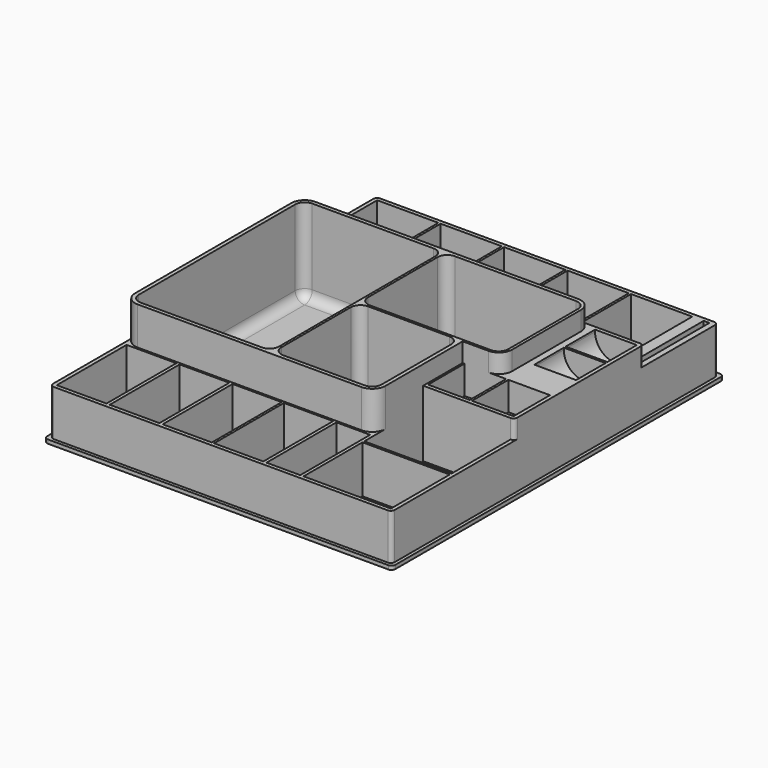
from build123d import *

# Parameters (mm, degrees)
F0_W      = 180
F0_H      = 215
F1_DEPTH  = 25
F2_W      = 166
F2_H      = 46
F2_W_2    = 53
F2_W_3    = 26.2
F2_W_4    = 46
F2_H_2    = 38.8
F2_W_5    = 52.9
F2_H_3    = 55.8
F2_W_6    = 45
F2_H_4    = 24
F2_W_7    = 22
F2_H_5    = 40
F2_W_8    = 73.9
F2_H_6    = 56
F2_H_7    = 113
F2_W_9    = 17.8
F2_W_10   = 3
F3_DEPTH  = 25.001
F4_W      = 180
F4_H      = 215
F5_DEPTH  = 1.2
F6_W      = 1.2
F6_H      = 46
F6_W_2    = 22
F6_H_2    = 1.2
F6_H_3    = 24
F7_DEPTH  = 25
F8_W      = 52.9
F8_H      = 55.8
F8_W_2    = 21.9
F8_H_2    = 24
F8_W_3    = 73.9
F8_H_3    = 113
F8_H_4    = 56
F8_W_4    = 22
F8_H_5    = 19.4
F9_DEPTH  = 20
F10_W     = 24
F10_H     = 20
F11_DEPTH = 45
F13_DEPTH = 40
F14_W     = 183.4
F14_H     = 218.4
F14_W_2   = 180
F14_H_2   = 215
F15_DEPTH = 2
F17_DEPTH = 10
F18_R     = 2
F19_R     = 5
F20_R     = 7


with BuildPart() as f1:
    # F0 (on Top) → F1 (new body)
    with BuildSketch(Plane.XY):
        with Locations((90, 107.5)):
            Rectangle(F0_W, F0_H)
    extrude(amount=F1_DEPTH)

    # F2 (on face) → F3 (cut, through all)
    with BuildSketch(Plane.XY.offset(25)):
        with Locations((85, 190)):
            Rectangle(F2_W, F2_H)
        with Locations((84.3, 25)):
            Rectangle(F2_W_2, F2_H)
        with Locations((15.1, 25)):
            Rectangle(F2_W_3, F2_H)
        with Locations((155, 21.4)):
            Rectangle(F2_W_4, F2_H_2)
        with Locations((155, 61.4)):
            Rectangle(F2_W_4, F2_H_2)
        with Locations((43, 25)):
            Rectangle(F2_W_3, F2_H)
        with Locations((103.55, 78.9)):
            Rectangle(F2_W_5, F2_H_3)
        with Locations((155.5, 94.8)):
            Rectangle(F2_W_6, F2_H_4)
        with Locations((167, 144)):
            Rectangle(F2_W_7, F2_H_5)
        with Locations((114.05, 136)):
            Rectangle(F2_W_8, F2_H_6)
        with Locations((38.95, 107.5)):
            Rectangle(F2_W_8, F2_H_7)
        with Locations((121.4, 25)):
            Rectangle(F2_W_9, F2_H)
        with Locations((175.5, 190)):
            Rectangle(F2_W_10, F2_H)
    extrude(amount=-F3_DEPTH, mode=Mode.SUBTRACT)

    # F4 (on Top) → F5 (join)
    with BuildSketch(Plane.XY):
        with Locations((90, 107.5)):
            Rectangle(F4_W, F4_H)
    extrude(amount=-F5_DEPTH)

    # F6 (on Top) → F7 (join, through all)
    with BuildSketch(Plane.XY):
        with Locations((34.84, 190)):
            Rectangle(F6_W, F6_H)
        with Locations((68.28, 190)):
            Rectangle(F6_W, F6_H)
        with Locations((101.72, 190)):
            Rectangle(F6_W, F6_H)
        with Locations((135.16, 190)):
            Rectangle(F6_W, F6_H)
        with Locations((84.3, 25)):
            Rectangle(F6_W, F6_H)
        with Locations((167, 144)):
            Rectangle(F6_W_2, F6_H_2)
        with Locations((155.5, 94.8)):
            Rectangle(F6_W, F6_H_3)
    extrude(amount=F7_DEPTH)

    # F8 (on face) → F9 (join)
    with BuildSketch(Plane.XY.offset(25)):
        Polygon((0, 166), (0, 49), (132, 49), (132, 80.8), (180, 80.8), (180, 166), (132, 166), align=None)
        with Locations((103.55, 78.9)):
            Rectangle(F8_W, F8_H, mode=Mode.SUBTRACT)
        with Locations((143.95, 94.8)):
            Rectangle(F8_W_2, F8_H_2, mode=Mode.SUBTRACT)
        with Locations((167.05, 94.8)):
            Rectangle(F8_W_2, F8_H_2, mode=Mode.SUBTRACT)
        with Locations((38.95, 107.5)):
            Rectangle(F8_W_3, F8_H_3, mode=Mode.SUBTRACT)
        with Locations((114.05, 136)):
            Rectangle(F8_W_3, F8_H_4, mode=Mode.SUBTRACT)
        with Locations((167, 133.7)):
            Rectangle(F8_W_4, F8_H_5, mode=Mode.SUBTRACT)
        with Locations((167, 154.3)):
            Rectangle(F8_W_4, F8_H_5, mode=Mode.SUBTRACT)
    extrude(amount=F9_DEPTH)

    # F10 (on face) → F11 (join, through all)
    with BuildSketch(Plane.YZ.offset(133)):
        with Locations((94.8, 10)):
            Rectangle(F10_W, F10_H)
    extrude(amount=F11_DEPTH)

    # F12 (on face) → F13 (join, through all)
    with BuildSketch(Plane.XZ.offset(-164)):
        with BuildLine():
            Line((156, 34), (156, 0))
            Line((156, 0), (178, 0))
            Line((178, 0), (178, 34))
            ThreePointArc((178, 34), (167, 23), (156, 34))
        make_face()
    extrude(amount=F13_DEPTH)

    # F14 (on face) → F15 (join)
    with BuildSketch(Plane(origin=(0, 0, -1.2), x_dir=(1, 0, 0), z_dir=(0, 0, -1))):
        with Locations((90, -107.5)):
            Rectangle(F14_W, F14_H)
        with Locations((90, -107.5)):
            Rectangle(F14_W_2, F14_H_2, mode=Mode.SUBTRACT)
    extrude(amount=-F15_DEPTH)

    # F16 (on face) → F17 (cut)
    with BuildSketch(Plane.XY.offset(45)):
        Polygon((132, 106.8), (132, 80.8), (180, 80.8), (180, 166), (152.5, 166), (152.5, 106.8), align=None)
    extrude(amount=-F17_DEPTH, mode=Mode.SUBTRACT)

    # F18
    f18_edges = [f1.edges().sort_by_distance(p)[0] for p in [
        (180, 0, 12.9),
        (180, 80.8, 30),
        (180, 166, 30),
        (180, 215, 12.9),
        (0, 215, 12.9),
        (0, 0, 12.9),
        (-1.7, -1.7, -0.2),
        (181.7, -1.7, -0.2),
        (181.7, 216.7, -0.2),
        (-1.7, 216.7, -0.2),
    ]]
    fillet(f18_edges, radius=F18_R)

    # F19
    f19_edges = [f1.edges().sort_by_distance(p)[0] for p in [
        (77.1, 78.9, 0),
        (103.55, 106.8, 0),
        (130, 78.9, 0),
        (103.55, 51, 0),
        (77.1, 136, 0),
        (114.05, 164, 0),
        (151, 136, 0),
        (114.05, 108, 0),
        (38.95, 164, 0),
        (75.9, 107.5, 0),
        (38.95, 51, 0),
        (2, 107.5, 0),
        (2, 51, 22.5),
        (2, 164, 22.5),
        (75.9, 164, 22.5),
        (75.9, 51, 22.5),
        (77.1, 106.8, 22.5),
        (77.1, 164, 22.5),
        (151, 164, 22.5),
        (151, 108, 22.5),
        (130, 106.8, 22.5),
        (130, 51, 22.5),
        (77.1, 51, 22.5),
        (77.1, 108, 22.5),
    ]]
    fillet(f19_edges, radius=F19_R)

    # F20
    f20_edges = [f1.edges().sort_by_distance(p)[0] for p in [
        (132, 49, 35),
        (0, 49, 35),
        (152.5, 106.8, 40),
        (152.5, 166, 40),
        (0, 166, 35),
    ]]
    fillet(f20_edges, radius=F20_R)


solid = f1.part
